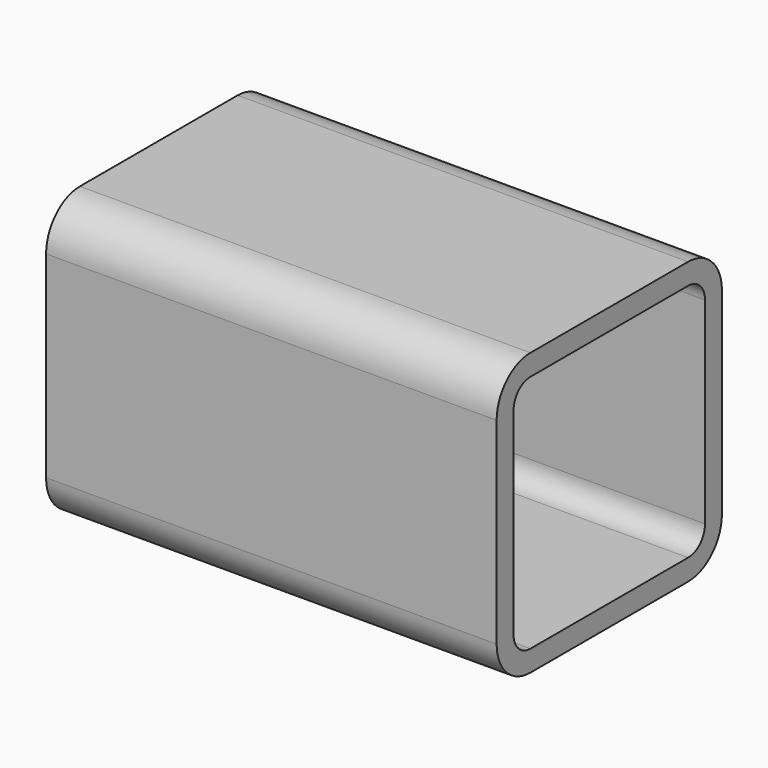
from build123d import *

# Parameters (mm, degrees)
F2_DEPTH = 101.6


# Not quite as in the source:
# - a variable given as a bare number and used for a length is read in inches; the dataset says mm whatever the document's units were


with BuildPart() as f2:
    # F1 (on Right) → F2 (new body, symmetric)
    with BuildSketch(Plane.YZ):
        with BuildLine():
            Line((44.45, 63.5), (-44.45, 63.5))
            ThreePointArc((-44.45, 63.5), (-57.9203841816, 57.9203841816), (-63.5, 44.45))
            Line((-63.5, 44.45), (-63.5, -44.45))
            ThreePointArc((-63.5, -44.45), (-57.9203841816, -57.9203841816), (-44.45, -63.5))
            Line((-44.45, -63.5), (44.45, -63.5))
            ThreePointArc((44.45, -63.5), (57.9203841816, -57.9203841816), (63.5, -44.45))
            Line((63.5, -44.45), (63.5, 44.45))
            ThreePointArc((63.5, 44.45), (57.9203841816, 57.9203841816), (44.45, 63.5))
        make_face()
        with BuildLine():
            ThreePointArc((-53.975, 44.45), (-51.1851920908, 51.1851920908), (-44.45, 53.975))
            Line((-44.45, 53.975), (44.45, 53.975))
            ThreePointArc((44.45, 53.975), (51.1851920908, 51.1851920908), (53.975, 44.45))
            Line((53.975, 44.45), (53.975, -44.45))
            ThreePointArc((53.975, -44.45), (51.1851920908, -51.1851920908), (44.45, -53.975))
            Line((44.45, -53.975), (-44.45, -53.975))
            ThreePointArc((-44.45, -53.975), (-51.1851920908, -51.1851920908), (-53.975, -44.45))
            Line((-53.975, -44.45), (-53.975, 44.45))
        make_face(mode=Mode.SUBTRACT)
    extrude(amount=F2_DEPTH, both=True)


solid = f2.part
